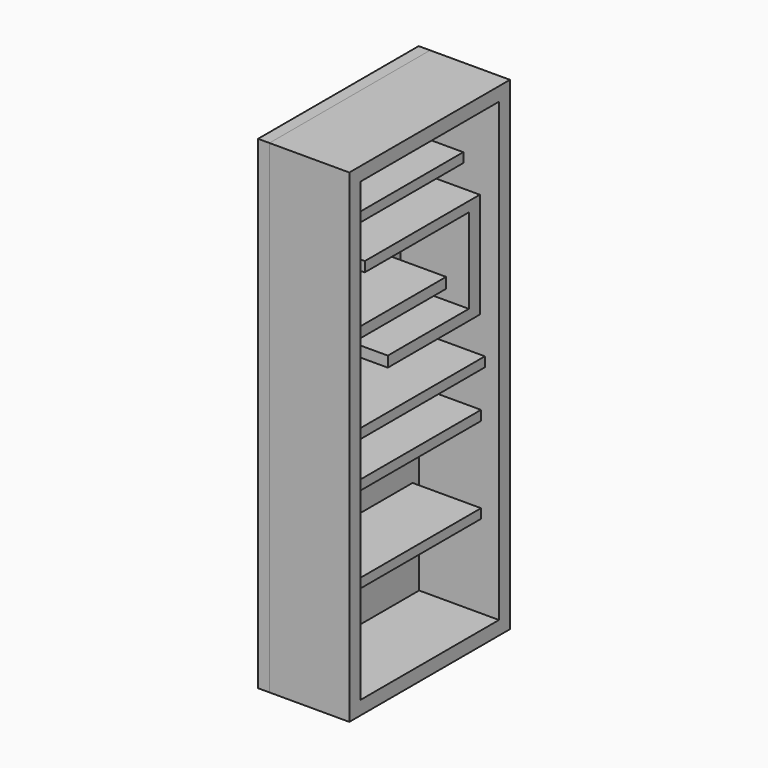
from build123d import *

# Parameters (mm, degrees)
F0_W     = 30
F0_H     = 1000
F1_DEPTH = 200
F0_W_2   = 380
F2_DEPTH = 25
F3_W     = 190
F3_H     = 1000
F4_DEPTH = 25
F5_W     = 293.8662618399
F5_H     = 21.023362875
F5_W_2   = 239.4576072693
F5_H_2   = 23.0258256197
F5_W_3   = 221.8910455704
F5_H_3   = 23.259088397
F5_W_4   = 348.6767783761
F5_H_4   = 21.4122384787
F5_W_5   = 350.4301086068
F5_H_5   = 20.5964148045
F6_DEPTH = 150
F7_W     = 346.3403731585
F7_H     = 21.2543550879
F8_DEPTH = 170


with BuildPart() as f1:
    # F0 (on Right) → F1 (new body)
    with BuildSketch(Plane.YZ):
        with Locations((-469.8110079765, -20.2939224243)):
            Rectangle(F0_W, F0_H)
        with Locations((-59.8110079765, -20.2939224243)):
            Rectangle(F0_W, F0_H)
        Polygon((-484.8110079765, 479.7060775757), (-454.8110079765, 479.7060775757), (-74.8110079765, 479.7060775757), (-44.8110079765, 479.7060775757), (-44.8110079765, 509.7060775757), (-484.8110079765, 509.7060775757), align=None)
        Polygon((-74.8110079765, -520.2939224243), (-454.8110079765, -520.2939224243), (-484.8110079765, -520.2939224243), (-484.8110079765, -550.2939224243), (-44.8110079765, -550.2939224243), (-44.8110079765, -520.2939224243), align=None)
    extrude(amount=F1_DEPTH)


with BuildPart() as f2:
    # F0 (on Right) → F2 (new body)
    with BuildSketch(Plane.YZ):
        with Locations((-59.8110079765, -20.2939224243)):
            Rectangle(F0_W, F0_H)
        Polygon((-484.8110079765, 479.7060775757), (-454.8110079765, 479.7060775757), (-74.8110079765, 479.7060775757), (-44.8110079765, 479.7060775757), (-44.8110079765, 509.7060775757), (-484.8110079765, 509.7060775757), align=None)
        Polygon((-74.8110079765, -520.2939224243), (-454.8110079765, -520.2939224243), (-484.8110079765, -520.2939224243), (-484.8110079765, -550.2939224243), (-44.8110079765, -550.2939224243), (-44.8110079765, -520.2939224243), align=None)
        with Locations((-469.8110079765, -20.2939224243)):
            Rectangle(F0_W, F0_H)
        with Locations((-264.8110079765, -20.2939224243)):
            Rectangle(F0_W_2, F0_H)
    extrude(amount=F2_DEPTH)

    # F5 (on face) → F6 (join)
    with BuildSketch(Plane.YZ.offset(25)):
        with Locations((-288.387157023, 390.7174617052)):
            Rectangle(F5_W, F5_H)
        Polygon((-96.1137637496, 300.7355630398), (-411.2088084221, 300.7355630398), (-411.2088084221, 278.9554297924), (-126.2423992157, 278.9554297924), (-96.1137637496, 278.9554297924), align=None)
        with Locations((-308.1502616405, 168.2250127196)):
            Rectangle(F5_W_2, F5_H_2)
        with Locations((-237.1879220009, 81.1184197664)):
            Rectangle(F5_W_3, F5_H_3)
        Polygon((-96.1137637496, 69.4888755679), (-96.1137637496, 278.9554297924), (-126.2423992157, 278.9554297924), (-126.2423992157, 92.7479639649), (-126.2423992157, 69.4888755679), align=None)
        with Locations((-267.1375088394, -126.4171227813)):
            Rectangle(F5_W_4, F5_H_4)
        with Locations((-268.0141739547, -315.7069832087)):
            Rectangle(F5_W_5, F5_H_5)
    extrude(amount=F6_DEPTH)

    # F7 (on face) → F8 (join)
    with BuildSketch(Plane.YZ.offset(25)):
        with Locations((-280.4818376899, -10.6271775439)):
            Rectangle(F7_W, F7_H)
    extrude(amount=F8_DEPTH)


with BuildPart() as f4:
    # F3 (on Right) → F4 (new body)
    with BuildSketch(Plane.YZ):
        with Locations((-361.7053023411, 4.1974354535)):
            Rectangle(F3_W, F3_H)
    extrude(amount=F4_DEPTH)


solid = Compound([f1.part, f2.part, f4.part])
